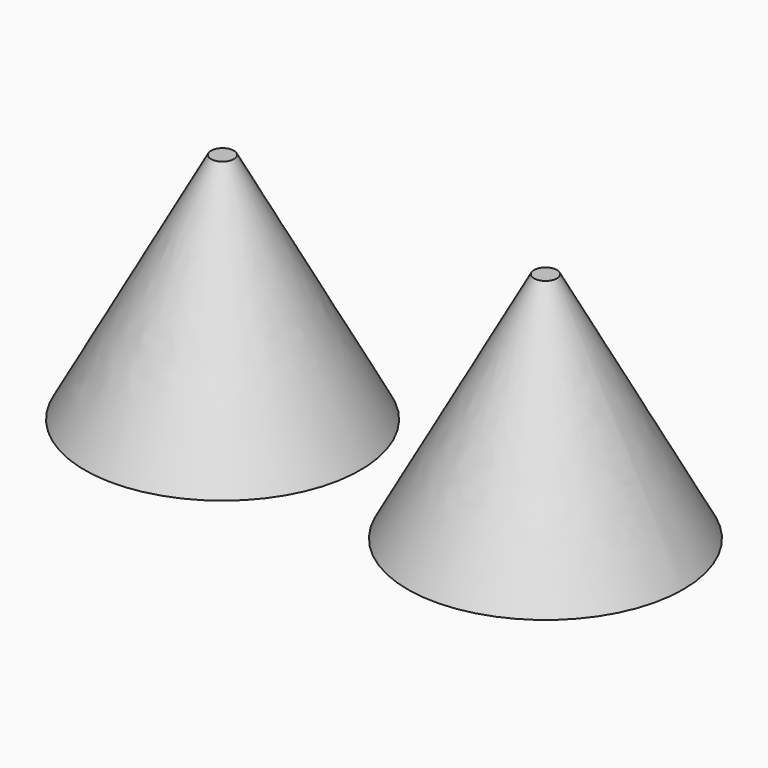
from build123d import *

# Parameters (mm, degrees)
F0_R = 30.1018278724
F3_R = 2.5001293044


with BuildPart() as f4:
    # F0 (on Top) → F4 section 0
    with BuildSketch(Plane.XY):
        with Locations((35.2490060031, 0)):
            Circle(F0_R)
    # F3 (on offset) → F4 section 1
    with BuildSketch(Plane.XY.offset(50.8)):
        with Locations((35.2580994368, 0)):
            Circle(F3_R)
    loft()


with BuildPart() as f5_1:
    # F5: instance of F4
    add(f4.part.mirror(Plane.YZ))


solid = Compound([f4.part, f5_1.part])
